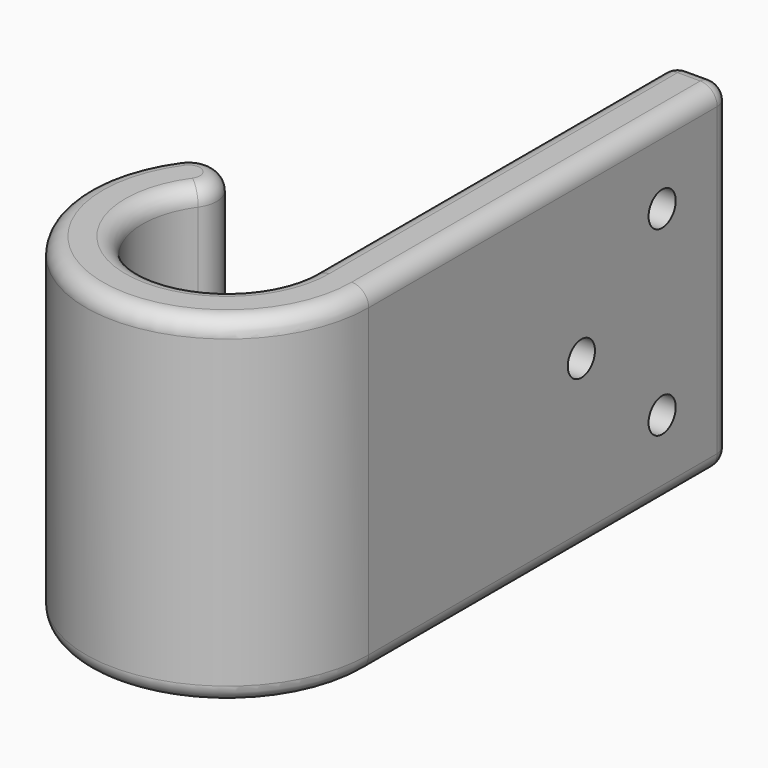
from build123d import *

# Parameters (mm, degrees)
F1_DEPTH      = 30
F2_R          = 1.5
F3_R          = 1.5
F4_DEPTH      = 25
F4_DEPTH_BACK = 25
F5_SIZE       = 2


# Not quite as in the source:
# - a feature names something its author has since deleted; it is built from what else it names


with BuildPart() as f1:
    # F0 (on Top) → F1 (new body)
    with BuildSketch(Plane.XY):
        with BuildLine():
            Line((-5, 40), (-5, 0))
            ThreePointArc((-5, 0), (-14.8093771881, -7.1355992743), (-18.5778072009, 4.3943440499))
            ThreePointArc((-18.5778072009, 4.3943440499), (-19.1389615845, 7.8850611335), (-22.6296786681, 7.3239067498))
            ThreePointArc((-22.6296786681, 7.3239067498), (-16.3489619801, -11.8926654572), (0, 0))
            Line((0, 0), (0, 40))
            Line((0, 40), (-5, 40))
        make_face()
    extrude(amount=F1_DEPTH)

    # F2
    f2_edges = [f1.edges().sort_by_distance(p)[0] for p in [
        (-5, 40, 15),
        (0, 40, 15),
        (-16.348962, -11.892665, 0),
        (-16.348962, -11.892665, 30),
        (0, 20, 0),
        (-14.809377, -7.135599, 0),
        (-14.809377, -7.135599, 30),
        (-5, 20, 0),
        (-18.577807, 4.394344, 15),
        (-5, 20, 30),
        (-2.5, 40, 0),
        (0, 0, 15),
        (-22.629679, 7.323907, 15),
        (-2.5, 40, 30),
        (0, 20, 30),
        (-19.138962, 7.885061, 0),
        (-19.138962, 7.885061, 30),
    ]]
    fillet(f2_edges, radius=F2_R)

    # F3 (on face) → F4 (cut, two sides)
    with BuildSketch(Plane(origin=(-5, 0, 0), x_dir=(0, -1, 0), z_dir=(-1, 0, 0))) as f4_sk:
        with Locations((-23.5, 15)):
            Circle(F3_R)
        with Locations((-32.419529755, 23.0275767795)):
            Circle(F3_R)
        with Locations((-32.419529755, 6.9724232205)):
            Circle(F3_R)
    extrude(amount=F4_DEPTH, mode=Mode.SUBTRACT)
    extrude(f4_sk.sketch, amount=-F4_DEPTH_BACK, mode=Mode.SUBTRACT)

    # F5
    f5_edges = [f1.edges().sort_by_distance(p)[0] for p in [
        (-5, 33.91953, 6.972423),
        (-5, 33.91953, 23.027577),
        (-5, 25, 15),
    ]]
    chamfer(f5_edges, length=F5_SIZE)


solid = f1.part
